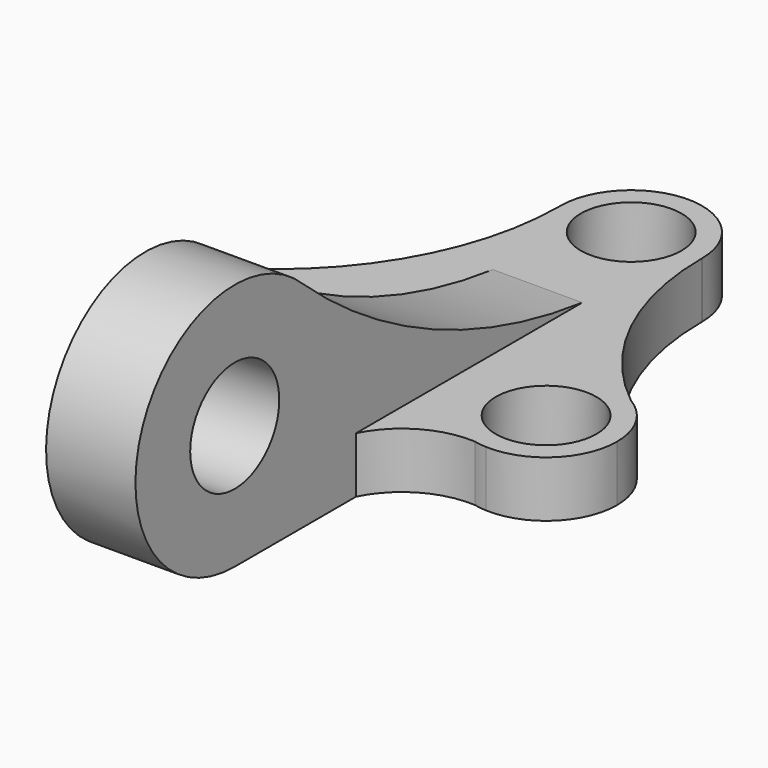
from build123d import *

# Parameters (mm, degrees)
F0_W     = 16.002
F0_H     = 11.1125
F1_DEPTH = 76.2
F0_R     = 9.017
F2_DEPTH = 10.0076
F3_R     = 9.9695
F4_DEPTH = 25.4


# Not quite as in the source:
# - a feature names something its author has since deleted; it is built from what else it names


with BuildPart() as f1:
    # F0 (on Top) → F1 (new body)
    with BuildSketch(Plane.XY):
        Polygon((-215.5320961376, 0), (-215.5320961376, 38.263771664), (-215.5320961376, 88.9), (-231.5340961376, 88.9), (-231.5340961376, 39.535600692), (-231.5340961376, 0), align=None)
        with Locations((-223.5330961376, -5.55625)):
            Rectangle(F0_W, F0_H)
    extrude(amount=F1_DEPTH)

    # F0 (on Top) → F2 (join)
    with BuildSketch(Plane.XY):
        with BuildLine():
            ThreePointArc((-210.8337106802, 109.7300639993), (-210.8332497742, 109.7925312439), (-210.8330961376, 109.855))
            ThreePointArc((-210.8330961376, 109.855), (-210.8331549592, 109.8936531274), (-210.8333314233, 109.9323058968))
            ThreePointArc((-210.8333314233, 109.9323058968), (-210.8336216962, 109.8311851368), (-210.8337106802, 109.7300639993))
        make_face()
        with BuildLine():
            ThreePointArc((-210.8337106802, 109.7300639993), (-210.8336216962, 109.8311851368), (-210.8333314233, 109.9323058968))
            ThreePointArc((-210.8333314233, 109.9323058968), (-223.438898877, 122.5546506596), (-236.2303167947, 110.12068324))
            ThreePointArc((-236.2303167947, 110.12068324), (-236.2290424274, 109.8342939205), (-236.229382634, 109.5479019679))
            ThreePointArc((-236.229382634, 109.5479019679), (-223.4420019429, 97.1553267031), (-210.8337106802, 109.7300639993))
        make_face()
        with Locations((-223.5330961376, 109.855)):
            Circle(F0_R, mode=Mode.SUBTRACT)
        with BuildLine():
            ThreePointArc((-191.660374853, 69.9817506227), (-205.7887196825, 87.6651452552), (-210.8337106802, 109.7300639993))
            ThreePointArc((-210.8337106802, 109.7300639993), (-223.4420019429, 97.1553267031), (-236.229382634, 109.5479019679))
            ThreePointArc((-236.229382634, 109.5479019679), (-241.3359242696, 87.5526791762), (-255.4702109751, 69.9433483413))
            ThreePointArc((-255.4702109751, 69.9433483413), (-242.6773531137, 70.1074060375), (-236.2330961376, 59.055))
            ThreePointArc((-236.2330961376, 59.055), (-238.6417428115, 51.6133572568), (-244.9540483765, 46.9944370399))
            ThreePointArc((-244.9540483765, 46.9944370399), (-237.2361698926, 45.078438676), (-231.5340961376, 39.535600692))
            Line((-231.5340961376, 39.535600692), (-231.5340961376, 88.9))
            Line((-231.5340961376, 88.9), (-215.5320961376, 88.9))
            Line((-215.5320961376, 88.9), (-215.5320961376, 38.263771664))
            ThreePointArc((-215.5320961376, 38.263771664), (-209.5064918471, 44.6635464864), (-200.94875069, 46.6710551745))
            ThreePointArc((-200.94875069, 46.6710551745), (-209.9310054796, 63.7559929971), (-191.660374853, 69.9817506227))
        make_face()
        with BuildLine():
            ThreePointArc((-236.229382634, 109.5479019679), (-236.2290424274, 109.8342939205), (-236.2303167947, 110.12068324))
            ThreePointArc((-236.2303167947, 110.12068324), (-236.2330792473, 109.8342873368), (-236.229382634, 109.5479019679))
        make_face()
        with BuildLine():
            ThreePointArc((-185.4330961376, 59.055), (-187.0992037982, 65.343339991), (-191.660374853, 69.9817506227))
            ThreePointArc((-191.660374853, 69.9817506227), (-209.9310054796, 63.7559929971), (-200.94875069, 46.6710551745))
            ThreePointArc((-200.94875069, 46.6710551745), (-199.8363704021, 46.5607848043), (-198.7350651606, 46.3692744277))
            ThreePointArc((-198.7350651606, 46.3692744277), (-189.3682517748, 49.8643796022), (-185.4330961376, 59.055))
        make_face()
        with Locations((-198.1330961376, 59.055)):
            Circle(F0_R, mode=Mode.SUBTRACT)
        with BuildLine():
            ThreePointArc((-257.5728060865, 68.3633517337), (-256.5112816453, 69.1397405149), (-255.4702109751, 69.9433483413))
            ThreePointArc((-255.4702109751, 69.9433483413), (-256.5625194428, 69.2079256882), (-257.5728060865, 68.3633517337))
        make_face()
        with BuildLine():
            ThreePointArc((-236.2330961376, 59.055), (-242.6773531137, 70.1074060375), (-255.4702109751, 69.9433483413))
            ThreePointArc((-255.4702109751, 69.9433483413), (-256.5112816453, 69.1397405149), (-257.5728060865, 68.3633517337))
            ThreePointArc((-257.5728060865, 68.3633517337), (-260.7702508926, 54.4537211227), (-249.0179411736, 46.3552834158))
            ThreePointArc((-249.0179411736, 46.3552834158), (-247.0076603385, 46.8126151022), (-244.9540483765, 46.9944370399))
            ThreePointArc((-244.9540483765, 46.9944370399), (-238.6417428115, 51.6133572568), (-236.2330961376, 59.055))
        make_face()
        with Locations((-248.9330961376, 59.055)):
            Circle(F0_R, mode=Mode.SUBTRACT)
        with BuildLine():
            ThreePointArc((-198.7350651606, 46.3692744277), (-199.8363704021, 46.5607848043), (-200.94875069, 46.6710551745))
            ThreePointArc((-200.94875069, 46.6710551745), (-199.8485569009, 46.4713918382), (-198.7350651606, 46.3692744277))
        make_face()
        Polygon((-215.5320961376, 0), (-215.5320961376, 38.263771664), (-215.5320961376, 88.9), (-231.5340961376, 88.9), (-231.5340961376, 39.535600692), (-231.5340961376, 0), align=None)
        with BuildLine():
            ThreePointArc((-249.0179411736, 46.3552834158), (-246.9599430632, 46.5092171649), (-244.9540483765, 46.9944370399))
            ThreePointArc((-244.9540483765, 46.9944370399), (-247.0076603385, 46.8126151022), (-249.0179411736, 46.3552834158))
        make_face()
        with Locations((-223.5330961376, -5.55625)):
            Rectangle(F0_W, F0_H)
    extrude(amount=F2_DEPTH)

    # F3 (on face) → F4 (cut)
    with BuildSketch(Plane(origin=(-231.5340961376, 0, 0), x_dir=(0, -1, 0), z_dir=(-1, 0, 0))):
        with BuildLine():
            ThreePointArc((-26.4295804615, 38.3289644541), (-2.3509786782, 42.6501406146), (11.1125, 22.225))
            Line((11.1125, 22.225), (11.1125, 76.2))
            Line((11.1125, 76.2), (-88.9, 76.2))
            Line((-88.9, 76.2), (-88.9, 10.0076))
            ThreePointArc((-88.9, 10.0076), (-55.490267729, 19.3717854622), (-26.4295804615, 38.3289644541))
        make_face()
        with Locations((-11.1125, 22.225)):
            Circle(F3_R)
        with BuildLine():
            Line((11.1125, 0), (11.1125, 22.225))
            ThreePointArc((11.1125, 22.225), (4.6029482119, 6.5095517881), (-11.1125, 0))
            Line((-11.1125, 0), (0, 0))
            Line((0, 0), (11.1125, 0))
        make_face()
    extrude(amount=-F4_DEPTH, mode=Mode.SUBTRACT)


solid = f1.part
